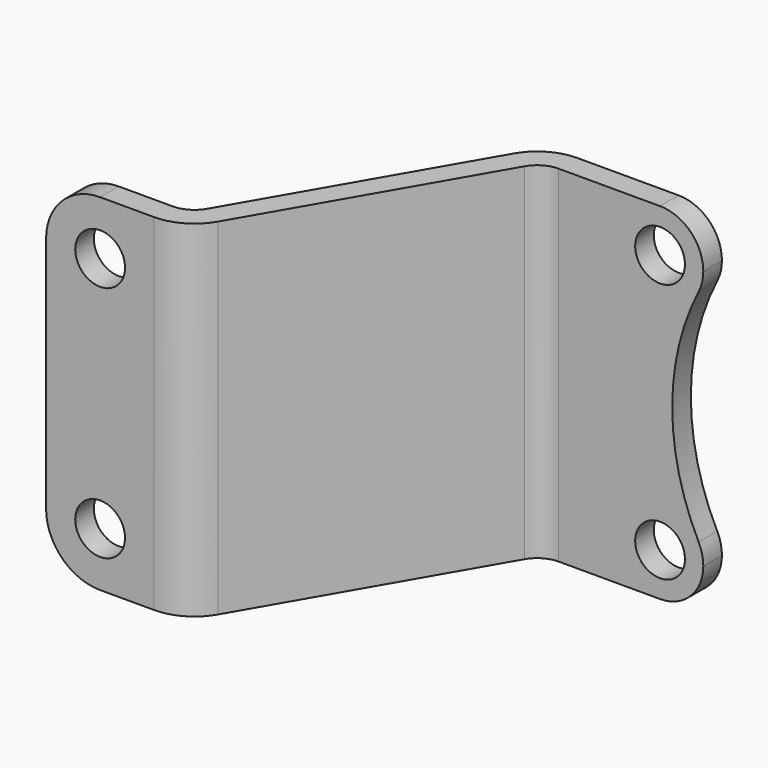
from build123d import *

# Parameters (mm, degrees)
F1_DEPTH = 25.4
F2_R     = 1.8288
F3_DEPTH = 1.70942
F4_R     = 1.98374
F5_R     = 3.69316
F6_R     = 3.17499
F7_R     = 3.96875
F8_R     = 1.8288
F9_DEPTH = 1.70942


# Not quite as in the source:
# - a fillet or chamfer is up to 0.001 mm smaller than in the source, because OpenCascade refuses the exact size


with BuildPart() as f1:
    # F0 (on Top) → F1 (new body)
    with BuildSketch(Plane.XY):
        Polygon((-10.0697469202, 0), (0, 0), (11.077711991, 19.18716), (22.839589814, 19.18716), (22.839589814, 20.89658), (10.0907778938, 20.89658), (-0.9869340972, 1.70942), (-10.0697469202, 1.70942), align=None)
    extrude(amount=F1_DEPTH)

    # F2 (on face) → F3 (cut, through all)
    with BuildSketch(Plane(origin=(0, 20.89658, 0), x_dir=(-1, 0, 0), z_dir=(0, 1, 0))):
        with BuildLine():
            ThreePointArc((-22.839589814, 3.175), (-22.752350863, 3.914159458), (-22.4954281104, 4.6126993912))
            ThreePointArc((-22.4954281104, 4.6126993912), (-20.5594607088, 12.7), (-22.4954281104, 20.7873006088))
            ThreePointArc((-22.4954281104, 20.7873006088), (-22.752350863, 21.485840542), (-22.839589814, 22.225))
            Line((-22.839589814, 22.225), (-22.839589814, 3.175))
        make_face()
        with Locations((-19.664589814, 3.175)):
            Circle(F2_R)
        with Locations((-19.664589814, 22.225)):
            Circle(F2_R)
    extrude(amount=-F3_DEPTH, mode=Mode.SUBTRACT)

    # F4
    f4_edges = [f1.edges().sort_by_distance(p)[0] for p in [
        (-0.986934, 1.70942, 12.7),
        (11.077712, 19.18716, 12.7),
    ]]
    fillet(f4_edges, radius=F4_R)

    # F5
    f5_edges = [f1.edges().sort_by_distance(p)[0] for p in [
        (10.090778, 20.89658, 12.7),
        (0, 0, 12.7),
    ]]
    fillet(f5_edges, radius=F5_R)

    # F6 (radius 3.175 in the source; OpenCascade refuses exactly that, so slightly less here)
    f6_edges = [f1.edges().sort_by_distance(p)[0] for p in [
        (22.83959, 20.04187, 25.4),
        (22.83959, 20.04187, 0),
    ]]
    fillet(f6_edges, radius=F6_R)

    # F7
    f7_edges = [f1.edges().sort_by_distance(p)[0] for p in [
        (-10.069747, 0.85471, 25.4),
        (-10.069747, 0.85471, 0),
    ]]
    fillet(f7_edges, radius=F7_R)

    # F8 (on face) → F9 (cut, through all)
    with BuildSketch(Plane(origin=(0, 1.70942, 0), x_dir=(-1, 0, 0), z_dir=(0, 1, 0))):
        with Locations((6.1009969202, 3.96875)):
            Circle(F8_R)
        with Locations((6.1009969202, 21.43125)):
            Circle(F8_R)
    extrude(amount=-F9_DEPTH, mode=Mode.SUBTRACT)


solid = f1.part
